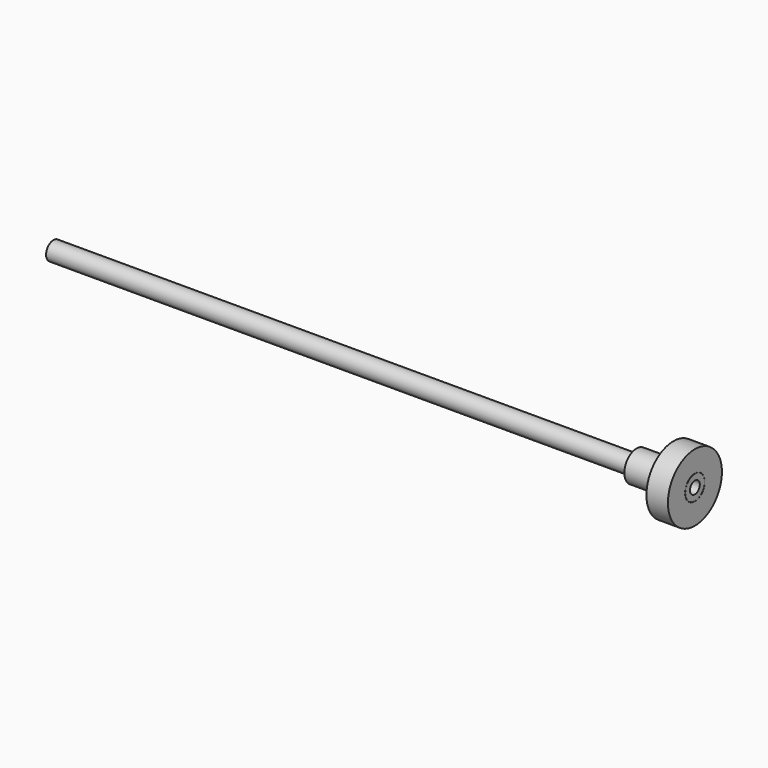
from build123d import *

# Parameters (mm, degrees)
F0_R     = 3
F1_DEPTH = 200
F2_R     = 5
F2_R_2   = 3
F2_R_3   = 2.95
F2_R_4   = 2
F3_DEPTH = 2
F4_DEPTH = 10
F5_R     = 3.95
F5_R_2   = 2
F6_DEPTH = 7
F7_R     = 11
F7_R_2   = 5
F7_R_3   = 4
F8_DEPTH = 7


with BuildPart() as f1:
    # F0 (on Right) → F1 (new body)
    with BuildSketch(Plane.YZ):
        Circle(F0_R)
    extrude(amount=F1_DEPTH)


with BuildPart() as f3:
    # F2 (on face) → F3 (new body)
    with BuildSketch(Plane.YZ.offset(200)):
        Circle(F2_R)
        Circle(F2_R_2, mode=Mode.SUBTRACT)
        Circle(F2_R_2)
        Circle(F2_R_3, mode=Mode.SUBTRACT)
        Circle(F2_R_3)
        Circle(F2_R_4, mode=Mode.SUBTRACT)
    extrude(amount=F3_DEPTH)

    # F2 (on face) → F4 (join)
    with BuildSketch(Plane.YZ.offset(200)):
        Circle(F2_R)
        Circle(F2_R_2, mode=Mode.SUBTRACT)
        Circle(F2_R_2)
        Circle(F2_R_3, mode=Mode.SUBTRACT)
    extrude(amount=-F4_DEPTH)

    # F5 (on face) → F6 (join)
    with BuildSketch(Plane.YZ.offset(202)):
        Circle(F5_R)
        Circle(F5_R_2, mode=Mode.SUBTRACT)
    extrude(amount=F6_DEPTH)


with BuildPart() as f8:
    # F7 (on face) → F8 (new body)
    with BuildSketch(Plane.YZ.offset(202)):
        Circle(F7_R)
        Circle(F7_R_2, mode=Mode.SUBTRACT)
        Circle(F7_R_2)
        Circle(F7_R_3, mode=Mode.SUBTRACT)
    extrude(amount=F8_DEPTH)


solid = Compound([f1.part, f3.part, f8.part])
